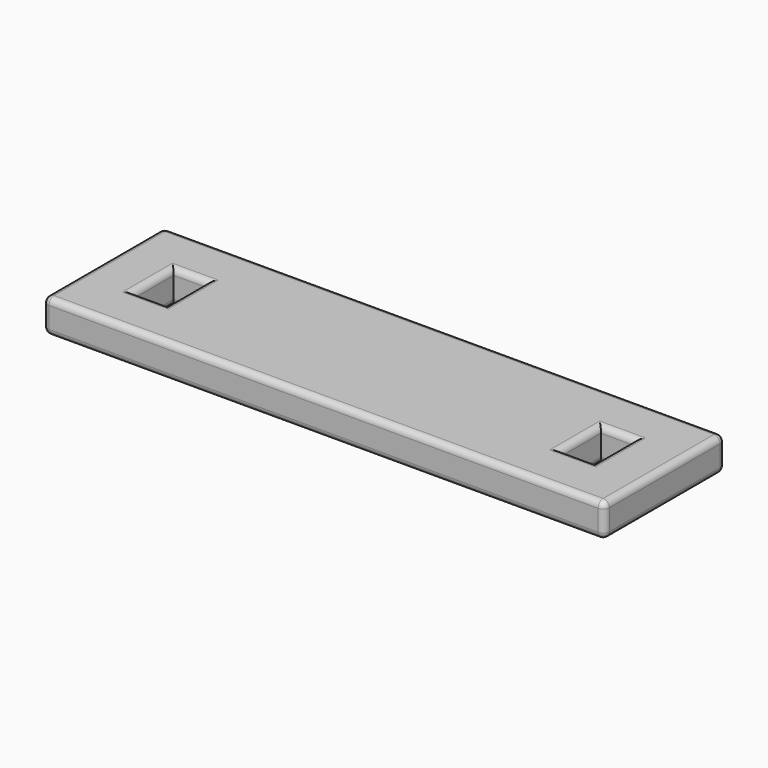
from build123d import *

# Parameters (mm, degrees)
F0_W          = 450
F0_H          = 121
F0_W_2        = 26.8
F0_H_2        = 40.2
F1_DEPTH      = 26.8
F2_R          = 5
F3_T1_DEPTH   = 440
F3_T3_DEPTH   = 111
F3_T5_DEPTH   = 40.2
F3_T7_DEPTH   = 26.8
F3_T9_DEPTH   = 26.8
F3_T11_DEPTH  = 16.8
F3_S15_W      = 5
F3_S15_H      = 5
F3_T16_DEPTH  = 5
F3_S21_W      = 5
F3_S21_H      = 5
F3_T22_DEPTH  = 5
F3_S27_W      = 5
F3_S27_H      = 5
F3_T28_DEPTH  = 5
F3_S33_W      = 5
F3_S33_H      = 5
F3_T34_DEPTH  = 5
F3_S39_W      = 5
F3_S39_H      = 5
F3_T40_DEPTH  = 5
F3_S45_W      = 5
F3_S45_H      = 5
F3_T46_DEPTH  = 5
F3_S51_W      = 5
F3_S51_H      = 5
F3_T52_DEPTH  = 5
F3_S57_W      = 5
F3_S57_H      = 5
F3_T58_DEPTH  = 5
F3_T65_DEPTH  = 39.3
F3_T69_DEPTH  = 52.7
F3_T76_DEPTH  = 39.3
F3_T80_DEPTH  = 52.7
F3_T87_DEPTH  = 39.3
F3_T91_DEPTH  = 52.7
F3_T98_DEPTH  = 52.7
F3_T102_DEPTH = 39.3
F3_T109_DEPTH = 52.7
F3_T113_DEPTH = 39.3
F3_T120_DEPTH = 52.7
F3_T124_DEPTH = 39.3
F3_T131_DEPTH = 52.7
F3_T135_DEPTH = 39.3
F3_T142_DEPTH = 39.3
F3_T146_DEPTH = 52.7


# Not quite as in the source:
# - a fillet or chamfer that OpenCascade refuses, or shapes differently, is made with other operations: its cross-section is extruded or revolved along the edge and cut away or added


with BuildPart() as f1:
    # F0 (on Top) → F1 (new body)
    with BuildSketch(Plane.XY):
        with Locations((-157.8, 57.318181593)):
            Rectangle(F0_W, F0_H)
        with Locations((-329, 57.318181593)):
            Rectangle(F0_W_2, F0_H_2, mode=Mode.SUBTRACT)
        with Locations((13.4, 57.318181593)):
            Rectangle(F0_W_2, F0_H_2, mode=Mode.SUBTRACT)
    extrude(amount=F1_DEPTH)

    # F2
    f2_edges = [f1.edges().sort_by_distance(p)[0] for p in [
        (67.2, 57.318182, 26.8),
        (-157.8, 117.818182, 26.8),
        (-382.8, 57.318182, 26.8),
        (-157.8, -3.181818, 26.8),
        (-342.4, 57.318182, 26.8),
        (-329, 77.418182, 26.8),
        (-315.6, 57.318182, 26.8),
        (-329, 37.218182, 26.8),
        (13.4, 77.418182, 26.8),
        (26.8, 57.318182, 26.8),
        (13.4, 37.218182, 26.8),
        (0, 57.318182, 26.8),
    ]]
    fillet(f2_edges, radius=F2_R)

    # F3: fillet of radius 5 on 16 edges, made by hand

    # F3_s2 → F3_t1 (cut)
    with BuildSketch(Plane.YZ.offset(-377.8)):
        with BuildLine():
            ThreePointArc((-3.181818407, 5), (-1.717352313, 1.4644660941), (1.818181593, 0))
            Line((1.818181593, 0), (-3.181818407, 0))
            Line((-3.181818407, 0), (-3.181818407, 5))
        make_face()
        with BuildLine():
            ThreePointArc((112.818181593, 0), (116.3537154989, 1.4644660941), (117.818181593, 5))
            Line((117.818181593, 5), (117.818181593, 0))
            Line((117.818181593, 0), (112.818181593, 0))
        make_face()
    extrude(amount=F3_T1_DEPTH, mode=Mode.SUBTRACT)

    # F3_s4 → F3_t3 (cut)
    with BuildSketch(Plane.XZ.offset(-112.818181593)):
        with BuildLine():
            ThreePointArc((-377.8, 0), (-381.3355339059, 1.4644660941), (-382.8, 5))
            Line((-382.8, 5), (-382.8, 0))
            Line((-382.8, 0), (-377.8, 0))
        make_face()
        with BuildLine():
            ThreePointArc((67.2, 5), (65.7355339059, 1.4644660941), (62.2, 0))
            Line((62.2, 0), (67.2, 0))
            Line((67.2, 0), (67.2, 5))
        make_face()
    extrude(amount=F3_T3_DEPTH, mode=Mode.SUBTRACT)

    # F3_s6 → F3_t5 (cut)
    with BuildSketch(Plane.XZ.offset(-77.418181593)):
        with BuildLine():
            ThreePointArc((-5, 0), (-1.4644660941, 1.4644660941), (0, 5))
            Line((0, 5), (0, 0))
            Line((0, 0), (-5, 0))
        make_face()
        with BuildLine():
            ThreePointArc((31.8, 0), (28.2644660941, 1.4644660941), (26.8, 5))
            Line((26.8, 5), (26.8, 0))
            Line((26.8, 0), (31.8, 0))
        make_face()
        with BuildLine():
            ThreePointArc((-347.4, 0), (-343.8644660941, 1.4644660941), (-342.4, 5))
            Line((-342.4, 5), (-342.4, 0))
            Line((-342.4, 0), (-347.4, 0))
        make_face()
        with BuildLine():
            ThreePointArc((-310.6, 0), (-314.1355339059, 1.4644660941), (-315.6, 5))
            Line((-315.6, 5), (-315.6, 0))
            Line((-315.6, 0), (-310.6, 0))
        make_face()
    extrude(amount=F3_T5_DEPTH, mode=Mode.SUBTRACT)

    # F3_s8 → F3_t7 (cut)
    with BuildSketch(Plane.YZ):
        with BuildLine():
            ThreePointArc((82.418181593, 0), (78.882647687, 1.4644660941), (77.418181593, 5))
            Line((77.418181593, 5), (77.418181593, 0))
            Line((77.418181593, 0), (82.418181593, 0))
        make_face()
        with BuildLine():
            ThreePointArc((32.218181593, 0), (35.7537154989, 1.4644660941), (37.218181593, 5))
            Line((37.218181593, 5), (37.218181593, 0))
            Line((37.218181593, 0), (32.218181593, 0))
        make_face()
    extrude(amount=F3_T7_DEPTH, mode=Mode.SUBTRACT)

    # F3_s10 → F3_t9 (cut)
    with BuildSketch(Plane.YZ.offset(-342.4)):
        with BuildLine():
            ThreePointArc((32.218181593, 0), (35.7537154989, 1.4644660941), (37.218181593, 5))
            Line((37.218181593, 5), (37.218181593, 0))
            Line((37.218181593, 0), (32.218181593, 0))
        make_face()
        with BuildLine():
            ThreePointArc((82.418181593, 0), (78.882647687, 1.4644660941), (77.418181593, 5))
            Line((77.418181593, 5), (77.418181593, 0))
            Line((77.418181593, 0), (82.418181593, 0))
        make_face()
    extrude(amount=F3_T9_DEPTH, mode=Mode.SUBTRACT)

    # F3_s12 → F3_t11 (cut)
    with BuildSketch(Plane.XY.offset(5)):
        with BuildLine():
            ThreePointArc((-377.8, -3.181818407), (-381.3355339059, -1.717352313), (-382.8, 1.818181593))
            Line((-382.8, 1.818181593), (-382.8, -3.181818407))
            Line((-382.8, -3.181818407), (-377.8, -3.181818407))
        make_face()
        with BuildLine():
            ThreePointArc((67.2, 1.818181593), (65.7355339059, -1.717352313), (62.2, -3.181818407))
            Line((62.2, -3.181818407), (67.2, -3.181818407))
            Line((67.2, -3.181818407), (67.2, 1.818181593))
        make_face()
        with BuildLine():
            ThreePointArc((-377.8, 117.818181593), (-381.3355339059, 116.3537154989), (-382.8, 112.818181593))
            Line((-382.8, 112.818181593), (-382.8, 117.818181593))
            Line((-382.8, 117.818181593), (-377.8, 117.818181593))
        make_face()
        with BuildLine():
            ThreePointArc((67.2, 112.818181593), (65.7355339059, 116.3537154989), (62.2, 117.818181593))
            Line((62.2, 117.818181593), (67.2, 117.818181593))
            Line((67.2, 117.818181593), (67.2, 112.818181593))
        make_face()
    extrude(amount=F3_T11_DEPTH, mode=Mode.SUBTRACT)


with BuildPart() as f3_tool14:
    # F3_s15 → F3_t16 (new body)
    with BuildSketch(Plane.YZ.offset(62.2)):
        with Locations((115.318181593, 24.3)):
            Rectangle(F3_S15_W, F3_S15_H)
    extrude(amount=F3_T16_DEPTH)

    # F3_s17 → F3_t18 (revolve, cut)
    with BuildSketch(Plane(origin=(62.2, 112.818181593, 21.8), x_dir=(0, -0.7071067812, -0.7071067812), z_dir=(0, -0.7071067812, 0.7071067812))):
        with BuildLine():
            ThreePointArc((0, -5), (5, 0), (0, 5))
            Line((0, 5), (0, -5))
        make_face()
    revolve(axis=Axis((62.2, 112.818181593, 21.8), (1, 0, 0)), mode=Mode.SUBTRACT)


with BuildPart() as f1_1:
    add(f1.part)

    # F3_t13: cut F3_tool14
    add(f3_tool14.part, mode=Mode.SUBTRACT)


with BuildPart() as f3_tool20:
    # F3_s21 → F3_t22 (new body)
    with BuildSketch(Plane.XZ.offset(-112.818181593)):
        with Locations((-380.3, 24.3)):
            Rectangle(F3_S21_W, F3_S21_H)
    extrude(amount=-F3_T22_DEPTH)

    # F3_s23 → F3_t24 (revolve, cut)
    with BuildSketch(Plane(origin=(-377.8, 112.818181593, 21.8), x_dir=(0.7071067812, 0, -0.7071067812), z_dir=(0.7071067812, 0, 0.7071067812))):
        with BuildLine():
            ThreePointArc((0, -5), (5, 0), (0, 5))
            Line((0, 5), (0, -5))
        make_face()
    revolve(axis=Axis((-377.8, 112.818181593, 21.8), (0, 1, 0)), mode=Mode.SUBTRACT)


with BuildPart() as f1_2:
    add(f1_1.part)

    # F3_t19: cut F3_tool20
    add(f3_tool20.part, mode=Mode.SUBTRACT)


with BuildPart() as f3_tool26:
    # F3_s27 → F3_t28 (new body)
    with BuildSketch(Plane.YZ.offset(62.2)):
        with Locations((-0.681818407, 24.3)):
            Rectangle(F3_S27_W, F3_S27_H)
    extrude(amount=F3_T28_DEPTH)

    # F3_s29 → F3_t30 (revolve, cut)
    with BuildSketch(Plane(origin=(62.2, 1.818181593, 21.8), x_dir=(0, 0.7071067812, -0.7071067812), z_dir=(0, -0.7071067812, -0.7071067812))):
        with BuildLine():
            ThreePointArc((0, -5), (5, 0), (0, 5))
            Line((0, 5), (0, -5))
        make_face()
    revolve(axis=Axis((62.2, 1.818181593, 21.8), (1, 0, 0)), mode=Mode.SUBTRACT)


with BuildPart() as f1_3:
    add(f1_2.part)

    # F3_t25: cut F3_tool26
    add(f3_tool26.part, mode=Mode.SUBTRACT)


with BuildPart() as f3_tool32:
    # F3_s33 → F3_t34 (new body)
    with BuildSketch(Plane.XZ.offset(-1.818181593)):
        with Locations((-380.3, 24.3)):
            Rectangle(F3_S33_W, F3_S33_H)
    extrude(amount=F3_T34_DEPTH)

    # F3_s35 → F3_t36 (revolve, cut)
    with BuildSketch(Plane(origin=(-377.8, 1.818181593, 21.8), x_dir=(0.7071067812, 0, -0.7071067812), z_dir=(-0.7071067812, 0, -0.7071067812))):
        with BuildLine():
            ThreePointArc((0, -5), (5, 0), (0, 5))
            Line((0, 5), (0, -5))
        make_face()
    revolve(axis=Axis((-377.8, 1.818181593, 21.8), (0, -1, 0)), mode=Mode.SUBTRACT)


with BuildPart() as f1_4:
    add(f1_3.part)

    # F3_t31: cut F3_tool32
    add(f3_tool32.part, mode=Mode.SUBTRACT)


with BuildPart() as f3_tool38:
    # F3_s39 → F3_t40 (new body)
    with BuildSketch(Plane.XZ.offset(-1.818181593)):
        with Locations((-380.3, 2.5)):
            Rectangle(F3_S39_W, F3_S39_H)
    extrude(amount=F3_T40_DEPTH)

    # F3_s41 → F3_t42 (revolve, cut)
    with BuildSketch(Plane(origin=(-377.8, 1.818181593, 5), x_dir=(0.7071067812, 0, 0.7071067812), z_dir=(0.7071067812, 0, -0.7071067812))):
        with BuildLine():
            ThreePointArc((0, -5), (5, 0), (0, 5))
            Line((0, 5), (0, -5))
        make_face()
    revolve(axis=Axis((-377.8, 1.818181593, 5), (0, -1, 0)), mode=Mode.SUBTRACT)


with BuildPart() as f1_5:
    add(f1_4.part)

    # F3_t37: cut F3_tool38
    add(f3_tool38.part, mode=Mode.SUBTRACT)


with BuildPart() as f3_tool44:
    # F3_s45 → F3_t46 (new body)
    with BuildSketch(Plane.YZ.offset(62.2)):
        with Locations((-0.681818407, 2.5)):
            Rectangle(F3_S45_W, F3_S45_H)
    extrude(amount=F3_T46_DEPTH)

    # F3_s47 → F3_t48 (revolve, cut)
    with BuildSketch(Plane(origin=(62.2, 1.818181593, 5), x_dir=(0, 0.7071067812, 0.7071067812), z_dir=(0, 0.7071067812, -0.7071067812))):
        with BuildLine():
            ThreePointArc((0, -5), (5, 0), (0, 5))
            Line((0, 5), (0, -5))
        make_face()
    revolve(axis=Axis((62.2, 1.818181593, 5), (1, 0, 0)), mode=Mode.SUBTRACT)


with BuildPart() as f1_6:
    add(f1_5.part)

    # F3_t43: cut F3_tool44
    add(f3_tool44.part, mode=Mode.SUBTRACT)


with BuildPart() as f3_tool50:
    # F3_s51 → F3_t52 (new body)
    with BuildSketch(Plane.XY.offset(5)):
        with Locations((-380.3, 115.318181593)):
            Rectangle(F3_S51_W, F3_S51_H)
    extrude(amount=-F3_T52_DEPTH)

    # F3_s53 → F3_t54 (revolve, cut)
    with BuildSketch(Plane(origin=(-377.8, 112.818181593, 5), x_dir=(0.7071067812, -0.7071067812, 0), z_dir=(0.7071067812, 0.7071067812, 0))):
        with BuildLine():
            ThreePointArc((0, -5), (5, 0), (0, 5))
            Line((0, 5), (0, -5))
        make_face()
    revolve(axis=Axis((-377.8, 112.818181593, 5), (0, 0, -1)), mode=Mode.SUBTRACT)


with BuildPart() as f1_7:
    add(f1_6.part)

    # F3_t49: cut F3_tool50
    add(f3_tool50.part, mode=Mode.SUBTRACT)


with BuildPart() as f3_tool56:
    # F3_s57 → F3_t58 (new body)
    with BuildSketch(Plane.YZ.offset(62.2)):
        with Locations((115.318181593, 2.5)):
            Rectangle(F3_S57_W, F3_S57_H)
    extrude(amount=F3_T58_DEPTH)

    # F3_s59 → F3_t60 (revolve, cut)
    with BuildSketch(Plane(origin=(62.2, 112.818181593, 5), x_dir=(0, -0.7071067812, 0.7071067812), z_dir=(0, 0.7071067812, 0.7071067812))):
        with BuildLine():
            ThreePointArc((0, -5), (5, 0), (0, 5))
            Line((0, 5), (0, -5))
        make_face()
    revolve(axis=Axis((62.2, 112.818181593, 5), (1, 0, 0)), mode=Mode.SUBTRACT)


with BuildPart() as f1_8:
    add(f1_7.part)

    # F3_t55: cut F3_tool56
    add(f3_tool56.part, mode=Mode.SUBTRACT)


with BuildPart() as f3_tool63:
    # F3_s64 → F3_t65 (new body)
    with BuildSketch(Plane.YZ.offset(26.8)):
        with BuildLine():
            ThreePointArc((32.218181593, 0), (35.7537154989, 1.4644660941), (37.218181593, 5))
            Line((37.218181593, 5), (37.218181593, 0))
            Line((37.218181593, 0), (32.218181593, 0))
        make_face()
    extrude(amount=-F3_T65_DEPTH)

    split(bisect_by=Plane.YZ, keep=Keep.BOTTOM)


with BuildPart() as f3_tool67:
    # F3_s68 → F3_t69 (new body)
    with BuildSketch(Plane.XZ.offset(-24.718181593)):
        with BuildLine():
            ThreePointArc((-5, 0), (-1.4644660941, 1.4644660941), (0, 5))
            Line((0, 5), (0, 0))
            Line((0, 0), (-5, 0))
        make_face()
    extrude(amount=-F3_T69_DEPTH)

    split(bisect_by=Plane.XZ.offset(-37.218181593), keep=Keep.TOP)


with BuildPart() as f3_tool63_1:
    add(f3_tool63.part)

    # F3_t71: intersect F3_tool67
    add(f3_tool67.part, mode=Mode.INTERSECT)


with BuildPart() as f1_9:
    add(f1_8.part)

    # F3_t61: cut F3_tool63
    add(f3_tool63_1.part, mode=Mode.SUBTRACT)


with BuildPart() as f3_tool74:
    # F3_s75 → F3_t76 (new body)
    with BuildSketch(Plane.YZ.offset(-12.5)):
        with BuildLine():
            ThreePointArc((82.418181593, 0), (78.882647687, 1.4644660941), (77.418181593, 5))
            Line((77.418181593, 5), (77.418181593, 0))
            Line((77.418181593, 0), (82.418181593, 0))
        make_face()
    extrude(amount=F3_T76_DEPTH)

    split(bisect_by=Plane.YZ, keep=Keep.BOTTOM)


with BuildPart() as f3_tool78:
    # F3_s79 → F3_t80 (new body)
    with BuildSketch(Plane.XZ.offset(-37.218181593)):
        with BuildLine():
            ThreePointArc((-5, 0), (-1.4644660941, 1.4644660941), (0, 5))
            Line((0, 5), (0, 0))
            Line((0, 0), (-5, 0))
        make_face()
    extrude(amount=-F3_T80_DEPTH)

    split(bisect_by=Plane.XZ.offset(-77.418181593), keep=Keep.BOTTOM)


with BuildPart() as f3_tool74_1:
    add(f3_tool74.part)

    # F3_t82: intersect F3_tool78
    add(f3_tool78.part, mode=Mode.INTERSECT)


with BuildPart() as f1_10:
    add(f1_9.part)

    # F3_t72: cut F3_tool74
    add(f3_tool74_1.part, mode=Mode.SUBTRACT)


with BuildPart() as f3_tool85:
    # F3_s86 → F3_t87 (new body)
    with BuildSketch(Plane.YZ):
        with BuildLine():
            ThreePointArc((82.418181593, 0), (78.882647687, 1.4644660941), (77.418181593, 5))
            Line((77.418181593, 5), (77.418181593, 0))
            Line((77.418181593, 0), (82.418181593, 0))
        make_face()
    extrude(amount=F3_T87_DEPTH)

    split(bisect_by=Plane.YZ.offset(26.8), keep=Keep.TOP)


with BuildPart() as f3_tool89:
    # F3_s90 → F3_t91 (new body)
    with BuildSketch(Plane.XZ.offset(-89.918181593)):
        with BuildLine():
            ThreePointArc((31.8, 0), (28.2644660941, 1.4644660941), (26.8, 5))
            Line((26.8, 5), (26.8, 0))
            Line((26.8, 0), (31.8, 0))
        make_face()
    extrude(amount=F3_T91_DEPTH)

    split(bisect_by=Plane.XZ.offset(-77.418181593), keep=Keep.BOTTOM)


with BuildPart() as f3_tool85_1:
    add(f3_tool85.part)

    # F3_t93: intersect F3_tool89
    add(f3_tool89.part, mode=Mode.INTERSECT)


with BuildPart() as f1_11:
    add(f1_10.part)

    # F3_t83: cut F3_tool85
    add(f3_tool85_1.part, mode=Mode.SUBTRACT)


with BuildPart() as f3_tool96:
    # F3_s97 → F3_t98 (new body)
    with BuildSketch(Plane.XZ.offset(-77.418181593)):
        with BuildLine():
            ThreePointArc((31.8, 0), (28.2644660941, 1.4644660941), (26.8, 5))
            Line((26.8, 5), (26.8, 0))
            Line((26.8, 0), (31.8, 0))
        make_face()
    extrude(amount=F3_T98_DEPTH)

    split(bisect_by=Plane.XZ.offset(-37.218181593), keep=Keep.TOP)


with BuildPart() as f3_tool100:
    # F3_s101 → F3_t102 (new body)
    with BuildSketch(Plane.YZ.offset(39.3)):
        with BuildLine():
            ThreePointArc((32.218181593, 0), (35.7537154989, 1.4644660941), (37.218181593, 5))
            Line((37.218181593, 5), (37.218181593, 0))
            Line((37.218181593, 0), (32.218181593, 0))
        make_face()
    extrude(amount=-F3_T102_DEPTH)

    split(bisect_by=Plane.YZ.offset(26.8), keep=Keep.TOP)


with BuildPart() as f3_tool96_1:
    add(f3_tool96.part)

    # F3_t104: intersect F3_tool100
    add(f3_tool100.part, mode=Mode.INTERSECT)


with BuildPart() as f1_12:
    add(f1_11.part)

    # F3_t94: cut F3_tool96
    add(f3_tool96_1.part, mode=Mode.SUBTRACT)


with BuildPart() as f3_tool107:
    # F3_s108 → F3_t109 (new body)
    with BuildSketch(Plane.XZ.offset(-77.418181593)):
        with BuildLine():
            ThreePointArc((-310.6, 0), (-314.1355339059, 1.4644660941), (-315.6, 5))
            Line((-315.6, 5), (-315.6, 0))
            Line((-315.6, 0), (-310.6, 0))
        make_face()
    extrude(amount=F3_T109_DEPTH)

    split(bisect_by=Plane.XZ.offset(-37.218181593), keep=Keep.TOP)


with BuildPart() as f3_tool111:
    # F3_s112 → F3_t113 (new body)
    with BuildSketch(Plane.YZ.offset(-303.1)):
        with BuildLine():
            ThreePointArc((32.218181593, 0), (35.7537154989, 1.4644660941), (37.218181593, 5))
            Line((37.218181593, 5), (37.218181593, 0))
            Line((37.218181593, 0), (32.218181593, 0))
        make_face()
    extrude(amount=-F3_T113_DEPTH)

    split(bisect_by=Plane.YZ.offset(-315.6), keep=Keep.TOP)


with BuildPart() as f3_tool107_1:
    add(f3_tool107.part)

    # F3_t115: intersect F3_tool111
    add(f3_tool111.part, mode=Mode.INTERSECT)


with BuildPart() as f1_13:
    add(f1_12.part)

    # F3_t105: cut F3_tool107
    add(f3_tool107_1.part, mode=Mode.SUBTRACT)


with BuildPart() as f3_tool118:
    # F3_s119 → F3_t120 (new body)
    with BuildSketch(Plane.XZ.offset(-24.718181593)):
        with BuildLine():
            ThreePointArc((-347.4, 0), (-343.8644660941, 1.4644660941), (-342.4, 5))
            Line((-342.4, 5), (-342.4, 0))
            Line((-342.4, 0), (-347.4, 0))
        make_face()
    extrude(amount=-F3_T120_DEPTH)

    split(bisect_by=Plane.XZ.offset(-37.218181593), keep=Keep.TOP)


with BuildPart() as f3_tool122:
    # F3_s123 → F3_t124 (new body)
    with BuildSketch(Plane.YZ.offset(-315.6)):
        with BuildLine():
            ThreePointArc((32.218181593, 0), (35.7537154989, 1.4644660941), (37.218181593, 5))
            Line((37.218181593, 5), (37.218181593, 0))
            Line((37.218181593, 0), (32.218181593, 0))
        make_face()
    extrude(amount=-F3_T124_DEPTH)

    split(bisect_by=Plane.YZ.offset(-342.4), keep=Keep.BOTTOM)


with BuildPart() as f3_tool118_1:
    add(f3_tool118.part)

    # F3_t126: intersect F3_tool122
    add(f3_tool122.part, mode=Mode.INTERSECT)


with BuildPart() as f1_14:
    add(f1_13.part)

    # F3_t116: cut F3_tool118
    add(f3_tool118_1.part, mode=Mode.SUBTRACT)


with BuildPart() as f3_tool129:
    # F3_s130 → F3_t131 (new body)
    with BuildSketch(Plane.XZ.offset(-37.218181593)):
        with BuildLine():
            ThreePointArc((-347.4, 0), (-343.8644660941, 1.4644660941), (-342.4, 5))
            Line((-342.4, 5), (-342.4, 0))
            Line((-342.4, 0), (-347.4, 0))
        make_face()
    extrude(amount=-F3_T131_DEPTH)

    split(bisect_by=Plane.XZ.offset(-77.418181593), keep=Keep.BOTTOM)


with BuildPart() as f3_tool133:
    # F3_s134 → F3_t135 (new body)
    with BuildSketch(Plane.YZ.offset(-354.9)):
        with BuildLine():
            ThreePointArc((82.418181593, 0), (78.882647687, 1.4644660941), (77.418181593, 5))
            Line((77.418181593, 5), (77.418181593, 0))
            Line((77.418181593, 0), (82.418181593, 0))
        make_face()
    extrude(amount=F3_T135_DEPTH)

    split(bisect_by=Plane.YZ.offset(-342.4), keep=Keep.BOTTOM)


with BuildPart() as f3_tool129_1:
    add(f3_tool129.part)

    # F3_t137: intersect F3_tool133
    add(f3_tool133.part, mode=Mode.INTERSECT)


with BuildPart() as f1_15:
    add(f1_14.part)

    # F3_t127: cut F3_tool129
    add(f3_tool129_1.part, mode=Mode.SUBTRACT)


with BuildPart() as f3_tool140:
    # F3_s141 → F3_t142 (new body)
    with BuildSketch(Plane.YZ.offset(-342.4)):
        with BuildLine():
            ThreePointArc((82.418181593, 0), (78.882647687, 1.4644660941), (77.418181593, 5))
            Line((77.418181593, 5), (77.418181593, 0))
            Line((77.418181593, 0), (82.418181593, 0))
        make_face()
    extrude(amount=F3_T142_DEPTH)

    split(bisect_by=Plane.YZ.offset(-315.6), keep=Keep.TOP)


with BuildPart() as f3_tool144:
    # F3_s145 → F3_t146 (new body)
    with BuildSketch(Plane.XZ.offset(-89.918181593)):
        with BuildLine():
            ThreePointArc((-310.6, 0), (-314.1355339059, 1.4644660941), (-315.6, 5))
            Line((-315.6, 5), (-315.6, 0))
            Line((-315.6, 0), (-310.6, 0))
        make_face()
    extrude(amount=F3_T146_DEPTH)

    split(bisect_by=Plane.XZ.offset(-77.418181593), keep=Keep.BOTTOM)


with BuildPart() as f3_tool140_1:
    add(f3_tool140.part)

    # F3_t148: intersect F3_tool144
    add(f3_tool144.part, mode=Mode.INTERSECT)


with BuildPart() as f1_16:
    add(f1_15.part)

    # F3_t138: cut F3_tool140
    add(f3_tool140_1.part, mode=Mode.SUBTRACT)


solid = f1_16.part
